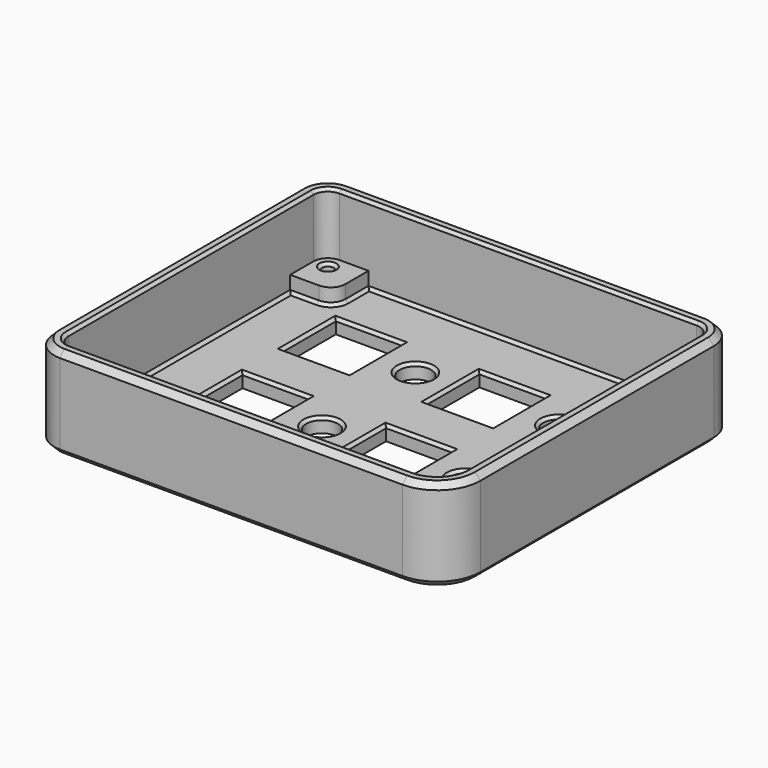
from build123d import *

# Parameters (mm, degrees)
F0_R     = 1
F1_DEPTH = 16
F2_T     = -2.5
F3_DEPTH = 5.3
F4_W     = 11.5
F4_H     = 11.5
F4_R     = 2.75
F4_W_2   = 41.64
F4_H_2   = 10.8
F5_DEPTH = 2.501
F6_SIZE  = 1
F7_SIZE  = 0.5


with BuildPart() as f1:
    # F0 (on Top) → F1 (new body)
    with BuildSketch(Plane.XY):
        with BuildLine():
            Line((26.035, -31.67), (28.575, -31.67))
            ThreePointArc((28.575, -31.67), (33.9065851301, -29.4615851301), (36.115, -24.13))
            Line((36.115, -24.13), (36.115, -21.59))
            Line((36.115, -21.59), (28.575, -21.59))
            ThreePointArc((28.575, -21.59), (26.7789487758, -22.3339487758), (26.035, -24.13))
            Line((26.035, -24.13), (26.035, -31.67))
        make_face()
        with Locations((28.575, -24.13)):
            Circle(F0_R, mode=Mode.SUBTRACT)
        with BuildLine():
            Line((-26.035, -31.67), (26.035, -31.67))
            Line((26.035, -31.67), (26.035, -24.13))
            ThreePointArc((26.035, -24.13), (26.7789487758, -22.3339487758), (28.575, -21.59))
            Line((28.575, -21.59), (36.115, -21.59))
            Line((36.115, -21.59), (36.115, 21.59))
            Line((36.115, 21.59), (28.575, 21.59))
            ThreePointArc((28.575, 21.59), (26.7789487758, 22.3339487758), (26.035, 24.13))
            Line((26.035, 24.13), (26.035, 31.67))
            Line((26.035, 31.67), (-26.035, 31.67))
            Line((-26.035, 31.67), (-26.035, 24.13))
            ThreePointArc((-26.035, 24.13), (-26.7789487758, 22.3339487758), (-28.575, 21.59))
            Line((-28.575, 21.59), (-36.115, 21.59))
            Line((-36.115, 21.59), (-36.115, -21.59))
            Line((-36.115, -21.59), (-28.575, -21.59))
            ThreePointArc((-28.575, -21.59), (-26.7789487758, -22.3339487758), (-26.035, -24.13))
            Line((-26.035, -24.13), (-26.035, -31.67))
        make_face()
        with BuildLine():
            Line((-31.115, -31.67), (-26.035, -31.67))
            Line((-26.035, -31.67), (-26.035, -24.13))
            ThreePointArc((-26.035, -24.13), (-26.7789487758, -22.3339487758), (-28.575, -21.59))
            Line((-28.575, -21.59), (-36.115, -21.59))
            Line((-36.115, -21.59), (-36.115, -26.67))
            ThreePointArc((-36.115, -26.67), (-34.6505339059, -30.2055339059), (-31.115, -31.67))
        make_face()
        with Locations((-31.115, -26.67)):
            Circle(F0_R, mode=Mode.SUBTRACT)
        with BuildLine():
            Line((-36.115, 26.67), (-36.115, 21.59))
            Line((-36.115, 21.59), (-28.575, 21.59))
            ThreePointArc((-28.575, 21.59), (-26.7789487758, 22.3339487758), (-26.035, 24.13))
            Line((-26.035, 24.13), (-26.035, 31.67))
            Line((-26.035, 31.67), (-31.115, 31.67))
            ThreePointArc((-31.115, 31.67), (-34.6505339059, 30.2055339059), (-36.115, 26.67))
        make_face()
        with Locations((-31.115, 26.67)):
            Circle(F0_R, mode=Mode.SUBTRACT)
        with BuildLine():
            Line((28.575, 21.59), (36.115, 21.59))
            Line((36.115, 21.59), (36.115, 26.67))
            ThreePointArc((36.115, 26.67), (34.6505339059, 30.2055339059), (31.115, 31.67))
            Line((31.115, 31.67), (26.035, 31.67))
            Line((26.035, 31.67), (26.035, 24.13))
            ThreePointArc((26.035, 24.13), (26.7789487758, 22.3339487758), (28.575, 21.59))
        make_face()
        with Locations((31.115, 26.67)):
            Circle(F0_R, mode=Mode.SUBTRACT)
        with Locations((31.115, 26.67)):
            Circle(F0_R)
        with Locations((-31.115, 26.67)):
            Circle(F0_R)
        with Locations((-31.115, -26.67)):
            Circle(F0_R)
        with Locations((28.575, -24.13)):
            Circle(F0_R)
    extrude(amount=F1_DEPTH)

    # F2
    f2_openings = [f1.faces().sort_by_distance(p)[0] for p in [
        (-0.051092, 0.04441, 16),
    ]]
    offset(amount=F2_T, openings=f2_openings)

    # F0 (on Top) → F3 (join)
    with BuildSketch(Plane.XY):
        with BuildLine():
            Line((-31.115, -31.67), (-26.035, -31.67))
            Line((-26.035, -31.67), (-26.035, -24.13))
            ThreePointArc((-26.035, -24.13), (-26.7789487758, -22.3339487758), (-28.575, -21.59))
            Line((-28.575, -21.59), (-36.115, -21.59))
            Line((-36.115, -21.59), (-36.115, -26.67))
            ThreePointArc((-36.115, -26.67), (-34.6505339059, -30.2055339059), (-31.115, -31.67))
        make_face()
        with Locations((-31.115, -26.67)):
            Circle(F0_R, mode=Mode.SUBTRACT)
        with BuildLine():
            Line((26.035, -31.67), (28.575, -31.67))
            ThreePointArc((28.575, -31.67), (33.9065851301, -29.4615851301), (36.115, -24.13))
            Line((36.115, -24.13), (36.115, -21.59))
            Line((36.115, -21.59), (28.575, -21.59))
            ThreePointArc((28.575, -21.59), (26.7789487758, -22.3339487758), (26.035, -24.13))
            Line((26.035, -24.13), (26.035, -31.67))
        make_face()
        with Locations((28.575, -24.13)):
            Circle(F0_R, mode=Mode.SUBTRACT)
        with BuildLine():
            Line((28.575, 21.59), (36.115, 21.59))
            Line((36.115, 21.59), (36.115, 26.67))
            ThreePointArc((36.115, 26.67), (34.6505339059, 30.2055339059), (31.115, 31.67))
            Line((31.115, 31.67), (26.035, 31.67))
            Line((26.035, 31.67), (26.035, 24.13))
            ThreePointArc((26.035, 24.13), (26.7789487758, 22.3339487758), (28.575, 21.59))
        make_face()
        with Locations((31.115, 26.67)):
            Circle(F0_R, mode=Mode.SUBTRACT)
        with BuildLine():
            Line((-36.115, 26.67), (-36.115, 21.59))
            Line((-36.115, 21.59), (-28.575, 21.59))
            ThreePointArc((-28.575, 21.59), (-26.7789487758, 22.3339487758), (-26.035, 24.13))
            Line((-26.035, 24.13), (-26.035, 31.67))
            Line((-26.035, 31.67), (-31.115, 31.67))
            ThreePointArc((-31.115, 31.67), (-34.6505339059, 30.2055339059), (-36.115, 26.67))
        make_face()
        with Locations((-31.115, 26.67)):
            Circle(F0_R, mode=Mode.SUBTRACT)
    extrude(amount=F3_DEPTH)

    # F4 (on face) → F5 (cut, through all)
    with BuildSketch(Plane.XY.offset(2.5)):
        with Locations((-18.415, 13.97)):
            Rectangle(F4_W, F4_H)
        with Locations((-18.415, -6.35)):
            Rectangle(F4_W, F4_H)
        with Locations((-5.715, 13.97)):
            Circle(F4_R)
        with Locations((-5.715, -6.35)):
            Circle(F4_R)
        with Locations((6.585, -6.35)):
            Rectangle(F4_W, F4_H)
        with Locations((6.585, 13.97)):
            Rectangle(F4_W, F4_H)
        with Locations((19.285, 13.97)):
            Circle(F4_R)
        with Locations((19.285, -6.35)):
            Circle(F4_R)
        with Locations((0.365, -21.42)):
            Rectangle(F4_W_2, F4_H_2)
    extrude(amount=-F5_DEPTH, mode=Mode.SUBTRACT)

    # F6
    f6_edges = [f1.edges().sort_by_distance(p)[0] for p in [
        (-36.115, 0, 16),
        (-34.650534, 30.205534, 16),
        (0, 31.67, 16),
        (34.650534, 30.205534, 16),
        (36.115, 1.27, 16),
        (33.906585, -29.461585, 16),
        (-1.27, -31.67, 16),
        (-34.650534, -30.205534, 0),
        (-34.650534, -30.205534, 16),
        (33.906585, -29.461585, 0),
        (-1.27, -31.67, 0),
        (36.115, 1.27, 0),
        (-36.115, 0, 0),
        (34.650534, 30.205534, 0),
        (-34.650534, 30.205534, 0),
        (0, 31.67, 0),
    ]]
    chamfer(f6_edges, length=F6_SIZE)

    # F7
    f7_edges = [f1.edges().sort_by_distance(p)[0] for p in [
        (-31.095, -21.59, 5.3),
        (-26.778949, -22.333949, 5.3),
        (-26.035, -26.65, 5.3),
        (-28.575, -29.17, 5.3),
        (-32.882767, -28.437767, 5.3),
        (-33.615, -24.13, 5.3),
        (-32.115, -26.67, 5.3),
        (31.095, -21.59, 2.5),
        (26.778949, -22.333949, 2.5),
        (33.615, 0, 2.5),
        (26.035, -26.65, 2.5),
        (31.095, 21.59, 2.5),
        (0, -29.17, 2.5),
        (26.778949, 22.333949, 2.5),
        (-26.035, -26.65, 2.5),
        (26.035, 26.65, 2.5),
        (-26.778949, -22.333949, 2.5),
        (0, 29.17, 2.5),
        (-31.095, -21.59, 2.5),
        (-26.035, 26.65, 2.5),
        (-33.615, 0, 2.5),
        (-26.778949, 22.333949, 2.5),
        (-31.095, 21.59, 2.5),
        (-24.165, -6.35, 2.5),
        (-18.415, -12.1, 2.5),
        (-12.665, -6.35, 2.5),
        (-18.415, -0.6, 2.5),
        (-8.465, -6.35, 2.5),
        (0.365, -16.02, 2.5),
        (-20.455, -21.42, 2.5),
        (0.365, -26.82, 2.5),
        (21.185, -21.42, 2.5),
        (0.835, -6.35, 2.5),
        (6.585, -12.1, 2.5),
        (12.335, -6.35, 2.5),
        (6.585, -0.6, 2.5),
        (16.535, -6.35, 2.5),
        (-18.415, 8.22, 2.5),
        (-12.665, 13.97, 2.5),
        (-18.415, 19.72, 2.5),
        (-24.165, 13.97, 2.5),
        (-8.465, 13.97, 2.5),
        (6.585, 8.22, 2.5),
        (12.335, 13.97, 2.5),
        (6.585, 19.72, 2.5),
        (0.835, 13.97, 2.5),
        (16.535, 13.97, 2.5),
        (-33.615, 0, 16),
        (-32.115, 26.67, 5.3),
        (0, 29.17, 16),
        (-32.882767, 28.437767, 16),
        (32.882767, 28.437767, 16),
        (30.115, 26.67, 5.3),
        (26.035, -26.65, 5.3),
        (26.778949, -22.333949, 5.3),
        (31.095, -21.59, 5.3),
        (33.615, -22.86, 5.3),
        (32.138818, -27.693818, 5.3),
        (27.305, -29.17, 5.3),
        (27.575, -24.13, 5.3),
        (32.138818, -27.693818, 16),
        (-1.27, -29.17, 16),
        (-32.882767, -28.437767, 16),
        (33.615, 1.27, 16),
        (-26.035, -29.17, 3.9),
        (26.035, -29.17, 3.9),
        (-33.615, -21.59, 3.9),
        (33.615, -21.59, 3.9),
    ]]
    chamfer(f7_edges, length=F7_SIZE)


solid = f1.part
